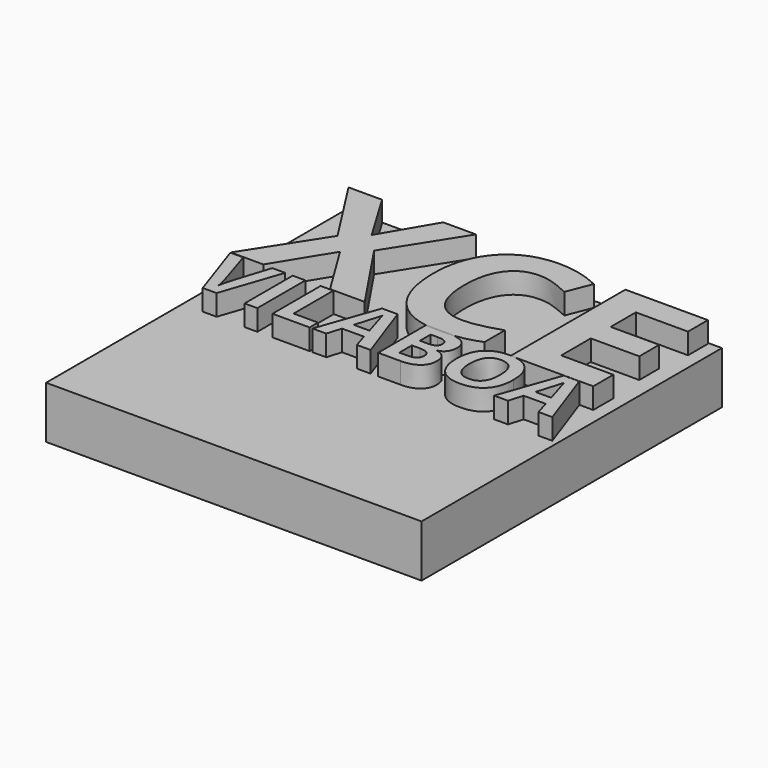
from build123d import *

# Parameters (mm, degrees)
F0_W         = 180
F0_H         = 180
F1_DEPTH     = 25
F2_TEXT_SIZE = 96.256684492
F3_DEPTH     = 10
F4_TEXT_SIZE = 40.3714736289
F5_DEPTH     = 10


# Not quite as in the source:
# - Text() gives the source's letters only with a copy of the font that has no kerning and outlines rounded to 1/6400 em; it was checked with that copy


with BuildPart() as f1:
    # F0 (on Top) → F1 (new body)
    with BuildSketch(Plane.XY):
        Rectangle(F0_W, F0_H)
    extrude(amount=F1_DEPTH)

    # F2 (on face) → F3 (join)
    with BuildSketch(Plane.XY.offset(25)):
        with Locations((-90, 20.6951871658)):
            Text('XCE', F2_TEXT_SIZE, font='Open Sans', font_style=FontStyle.BOLD, text_align=(TextAlign.LEFT, TextAlign.BOTTOM))
    extrude(amount=F3_DEPTH)

    # F4 (on face) → F5 (join)
    with BuildSketch(Plane.XY.offset(25)):
        with Locations((-90, -8.372273847)):
            Text('VILABOA', F4_TEXT_SIZE, font='Open Sans', font_style=FontStyle.BOLD, text_align=(TextAlign.LEFT, TextAlign.BOTTOM))
    extrude(amount=F5_DEPTH)


solid = f1.part
